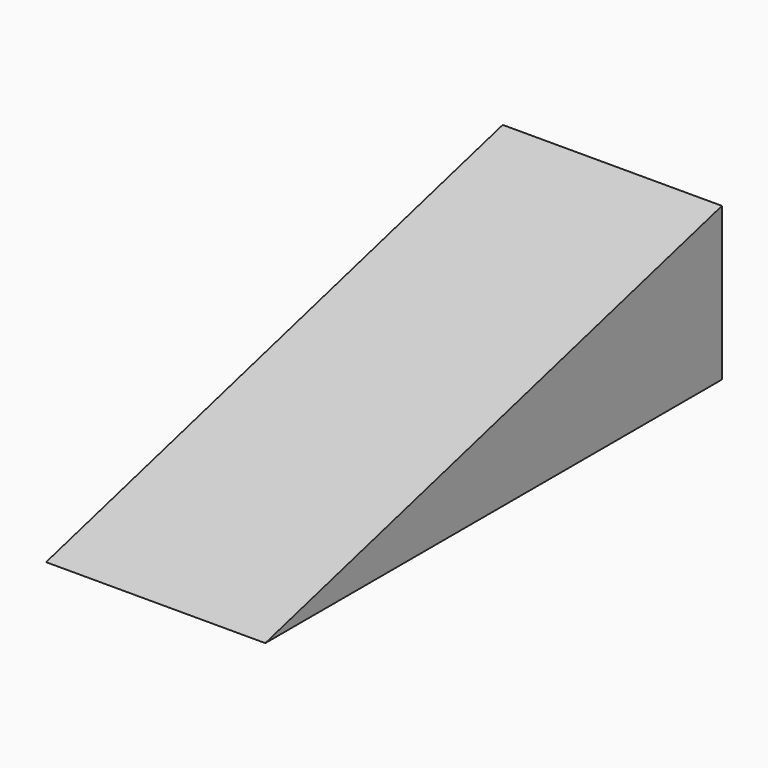
from build123d import *

# Parameters (mm, degrees)
F0_W        = 29.4894
F0_H        = 79.6798
F1_DEPTH    = 20.574
F2_T1_DEPTH = 443.3019107385
F3_T        = -2.54


# Not quite as in the source:
# - a fillet or chamfer that OpenCascade refuses, or shapes differently, is made with other operations: its cross-section is extruded or revolved along the edge and cut away or added


with BuildPart() as f1:
    # F0 (on Top) → F1 (new body)
    with BuildSketch(Plane.XY):
        with Locations((-15.601075187, 5.9804012012)):
            Rectangle(F0_W, F0_H)
    extrude(amount=F1_DEPTH)

    # F2: chamfer of 79.6798 x 21.3501380631 on 1 edges, made by hand

    # F2_s2 → F2_t1 (cut)
    with BuildSketch(Plane.YZ.offset(-237.2520305563)):
        Polygon((-33.8594987988, -0.7761380631), (45.8203012012, 20.574), (-33.8594987988, 20.574), align=None)
    extrude(amount=F2_T1_DEPTH, mode=Mode.SUBTRACT)

    # F3
    f3_openings = [f1.faces().sort_by_distance(p)[0] for p in [
        (-15.601075, 7.428695, 0),
    ]]
    offset(amount=F3_T, openings=f3_openings, kind=Kind.INTERSECTION)


solid = f1.part
